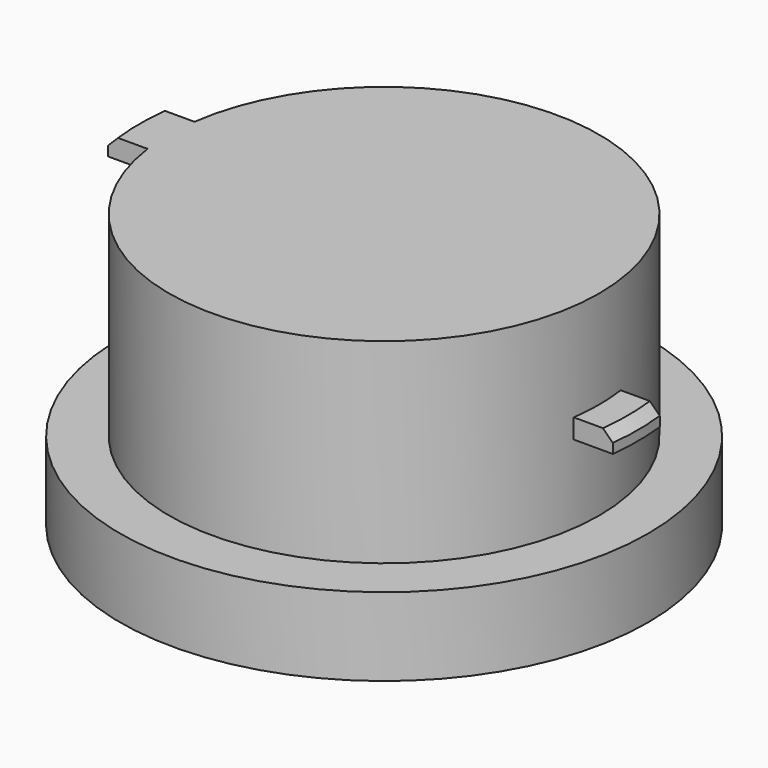
from build123d import *

# Parameters (mm, degrees)
F0_R          = 13.5
F1_DEPTH      = 4
F2_R          = 11
F3_DEPTH      = 10
F5_DEPTH      = 1
F8_DEPTH      = 1
F9_SIZE       = 0.5
F10_TEXT_SIZE = 5.4001753054
F11_DEPTH     = 1


# Not quite as in the source:
# - Text() gives the source's letters only with a copy of the font that has no kerning and outlines rounded to 1/6400 em; it was checked with that copy


with BuildPart() as f1:
    # F0 (on Top) → F1 (new body)
    with BuildSketch(Plane.XY):
        Circle(F0_R)
    extrude(amount=F1_DEPTH)

    # F2 (on face) → F3 (join)
    with BuildSketch(Plane.XY.offset(4)):
        Circle(F2_R)
    extrude(amount=F3_DEPTH)

    # F4 (on face) → F5 (join)
    with BuildSketch(Plane.XY.offset(14)):
        with BuildLine():
            Line((-10.8972473589, 1.5), (-12.9131715701, 1.5))
            ThreePointArc((-12.9131715701, 1.5), (-13, 0), (-12.9131715701, -1.5))
            Line((-12.9131715701, -1.5), (-10.8972473589, -1.5))
            ThreePointArc((-10.8972473589, -1.5), (-11, 0), (-10.8972473589, 1.5))
        make_face()
    extrude(amount=-F5_DEPTH)

    # F7 (on offset) → F8 (join)
    with BuildSketch(Plane.XY.offset(8)):
        with BuildLine():
            Line((10.8972473589, -1.5), (12.8972473589, -1.5))
            ThreePointArc((12.8972473589, -1.5), (12.9841822783, 0), (12.8972473589, 1.5))
            Line((12.8972473589, 1.5), (10.8972473589, 1.5))
            ThreePointArc((10.8972473589, 1.5), (11, 0), (10.8972473589, -1.5))
        make_face()
    extrude(amount=F8_DEPTH)

    # F9
    f9_edges = [f1.edges().sort_by_distance(p)[0] for p in [
        (-13, 0, 14),
        (12.984182, 0, 9),
    ]]
    chamfer(f9_edges, length=F9_SIZE)

    # F10 (on face) → F11 (cut)
    with BuildSketch(Plane(origin=(0, 0, 0), x_dir=(1, 0, 0), z_dir=(0, 0, -1))):
        with Locations((-7.9876007512, 2.5258020132)):
            Text("You're", F10_TEXT_SIZE, font='Open Sans', text_align=(TextAlign.LEFT, TextAlign.BOTTOM))
        with Locations((-7.9876007512, -4.8184364021)):
            Text('Grape!', F10_TEXT_SIZE, font='Open Sans', text_align=(TextAlign.LEFT, TextAlign.BOTTOM))
    extrude(amount=-F11_DEPTH, mode=Mode.SUBTRACT)


solid = f1.part
